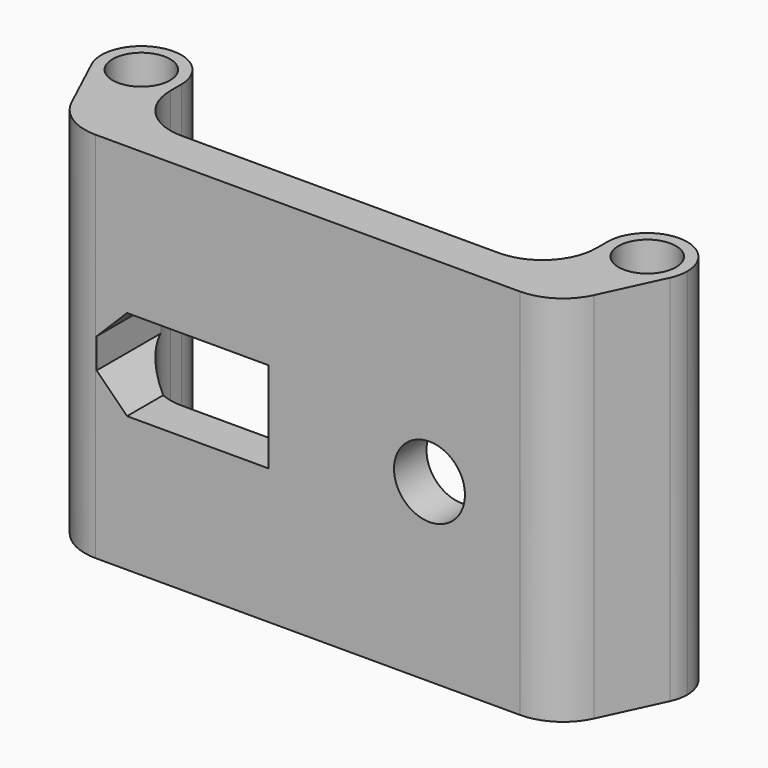
from build123d import *

# Parameters (mm, degrees)
F0_R         = 2.7
F1_DEPTH     = 35
F2_R         = 3.33
F3_DEPTH     = 13.911
F4_T1_DEPTH  = 35
F4_T6_DEPTH  = 47.7
F4_T11_DEPTH = 60.4
F4_T17_DEPTH = 47.7
F4_T23_DEPTH = 47.7
F4_T28_DEPTH = 60.4
F5_R         = 5.08


# Not quite as in the source:
# - a fillet or chamfer that OpenCascade refuses, or shapes differently, is made with other operations: its cross-section is extruded or revolved along the edge and cut away or added


with BuildPart() as f1:
    # F0 (on Top) → F1 (new body)
    with BuildSketch(Plane.XY):
        with BuildLine():
            Line((-20, -6.35), (-20, 0))
            ThreePointArc((-20, 0), (-22.9383514477, -3.6611100267), (-27.1486542014, -1.5848184815))
            Line((-27.1486542014, -1.5848184815), (-23.1499813893, -10.16))
            Line((-23.1499813893, -10.16), (23.1499813893, -10.16))
            Line((23.1499813893, -10.16), (27.1486542014, -1.5848184815))
            ThreePointArc((27.1486542014, -1.5848184815), (22.9383514477, -3.6611100267), (20, 0))
            Line((20, 0), (20, -6.35))
            Line((20, -6.35), (-20, -6.35))
        make_face()
        with BuildLine():
            ThreePointArc((-27.1486542014, -1.5848184815), (-22.9383514477, -3.6611100267), (-20, 0))
            ThreePointArc((-20, 0), (-24.5616485523, 3.6611100267), (-27.1486542014, -1.5848184815))
        make_face()
        with Locations((-23.75, 0)):
            Circle(F0_R, mode=Mode.SUBTRACT)
        with BuildLine():
            ThreePointArc((27.5, 0), (23.75, 3.75), (20, 0))
            ThreePointArc((20, 0), (22.9383514477, -3.6611100267), (27.1486542014, -1.5848184815))
            ThreePointArc((27.1486542014, -1.5848184815), (27.4111100267, -0.8116485523), (27.5, 0))
        make_face()
        with Locations((23.75, 0)):
            Circle(F0_R, mode=Mode.SUBTRACT)
    extrude(amount=F1_DEPTH)

    # F2 (on face) → F3 (cut, through all)
    with BuildSketch(Plane.XZ.offset(10.16)):
        Polygon((-3.683, 12.7), (-3.683, 21.228), (-16.9683, 21.228), (-19.8183, 18.378), (-19.8183, 15.55), (-16.9683, 12.7), align=None)
        with Locations((11.43, 16.51)):
            Circle(F2_R)
    extrude(amount=-F3_DEPTH, mode=Mode.SUBTRACT)

    # F4: fillet of radius 5.08 on 2 edges, made by hand

    # F4_s2 → F4_t1 (join)
    with BuildSketch(Plane.XY):
        with BuildLine():
            ThreePointArc((20, -1.27), (18.5121024484, -4.8621024484), (14.92, -6.35))
            Line((14.92, -6.35), (20, -6.35))
            Line((20, -6.35), (20, -1.27))
        make_face()
    extrude(amount=F4_T1_DEPTH)


with BuildPart() as f4_tool4:
    # F4_s5 → F4_t6 (new body)
    with BuildSketch(Plane.XY):
        with BuildLine():
            ThreePointArc((-14.92, -6.35), (-18.5121024484, -4.8621024484), (-20, -1.27))
            Line((-20, -1.27), (-20, -6.35))
            Line((-20, -6.35), (-14.92, -6.35))
        make_face()
    extrude(amount=F4_T6_DEPTH)

    split(bisect_by=Plane(origin=(-2.13415, 0, -2.13415), x_dir=(0, 1, 0), z_dir=(-0.7071067812, 0, -0.7071067812)), keep=Keep.TOP)


with BuildPart() as f1_1:
    add(f1.part)

    # F4_t3: union F4_tool4
    add(f4_tool4.part)


with BuildPart() as f4_tool9:
    # F4_s10 → F4_t11 (new body)
    with BuildSketch(Plane.XY.offset(-12.7)):
        with BuildLine():
            ThreePointArc((-14.92, -6.35), (-18.5121024484, -4.8621024484), (-20, -1.27))
            Line((-20, -1.27), (-20, -6.35))
            Line((-20, -6.35), (-14.92, -6.35))
        make_face()
    extrude(amount=F4_T11_DEPTH)

    split(bisect_by=Plane.XY.offset(12.7), keep=Keep.BOTTOM)

    split(bisect_by=Plane(origin=(-2.13415, 0, -2.13415), x_dir=(0, 1, 0), z_dir=(0.7071067812, 0, 0.7071067812)), keep=Keep.TOP)


with BuildPart() as f1_2:
    add(f1_1.part)

    # F4_t8: union F4_tool9
    add(f4_tool9.part)


with BuildPart() as f4_tool15:
    # F4_s16 → F4_t17 (new body)
    with BuildSketch(Plane.XY.offset(-12.7)):
        with BuildLine():
            ThreePointArc((-14.92, -6.35), (-18.5121024484, -4.8621024484), (-20, -1.27))
            Line((-20, -1.27), (-20, -6.35))
            Line((-20, -6.35), (-14.92, -6.35))
        make_face()
    extrude(amount=F4_T17_DEPTH)

    split(bisect_by=Plane(origin=(-2.13415, 0, -2.13415), x_dir=(0, 1, 0), z_dir=(0.7071067812, 0, 0.7071067812)), keep=Keep.TOP)

    split(bisect_by=Plane.YZ.offset(-19.8183), keep=Keep.BOTTOM)


with BuildPart() as f1_3:
    add(f1_2.part)

    # F4_t14: union F4_tool15
    add(f4_tool15.part)


with BuildPart() as f4_tool21:
    # F4_s22 → F4_t23 (new body)
    with BuildSketch(Plane.XY.offset(-12.7)):
        with BuildLine():
            ThreePointArc((-14.92, -6.35), (-18.5121024484, -4.8621024484), (-20, -1.27))
            Line((-20, -1.27), (-20, -6.35))
            Line((-20, -6.35), (-14.92, -6.35))
        make_face()
    extrude(amount=F4_T23_DEPTH)

    split(bisect_by=Plane(origin=(-19.09815, 0, 19.09815), x_dir=(0, 1, 0), z_dir=(-0.7071067812, 0, 0.7071067812)), keep=Keep.TOP)


with BuildPart() as f1_4:
    add(f1_3.part)

    # F4_t20: union F4_tool21
    add(f4_tool21.part)


with BuildPart() as f4_tool26:
    # F4_s27 → F4_t28 (new body)
    with BuildSketch(Plane.XY.offset(-12.7)):
        with BuildLine():
            ThreePointArc((-14.92, -6.35), (-18.5121024484, -4.8621024484), (-20, -1.27))
            Line((-20, -1.27), (-20, -6.35))
            Line((-20, -6.35), (-14.92, -6.35))
        make_face()
    extrude(amount=F4_T28_DEPTH)

    split(bisect_by=Plane(origin=(-19.09815, 0, 19.09815), x_dir=(0, 1, 0), z_dir=(0.7071067812, 0, -0.7071067812)), keep=Keep.TOP)

    split(bisect_by=Plane.XY.offset(21.228), keep=Keep.TOP)


with BuildPart() as f1_5:
    add(f1_4.part)

    # F4_t25: union F4_tool26
    add(f4_tool26.part)

    # F5
    f5_edges = [f1_5.edges().sort_by_distance(p)[0] for p in [
        (-23.149981, -10.16, 17.5),
        (23.149981, -10.16, 17.5),
    ]]
    fillet(f5_edges, radius=F5_R)


solid = f1_5.part
